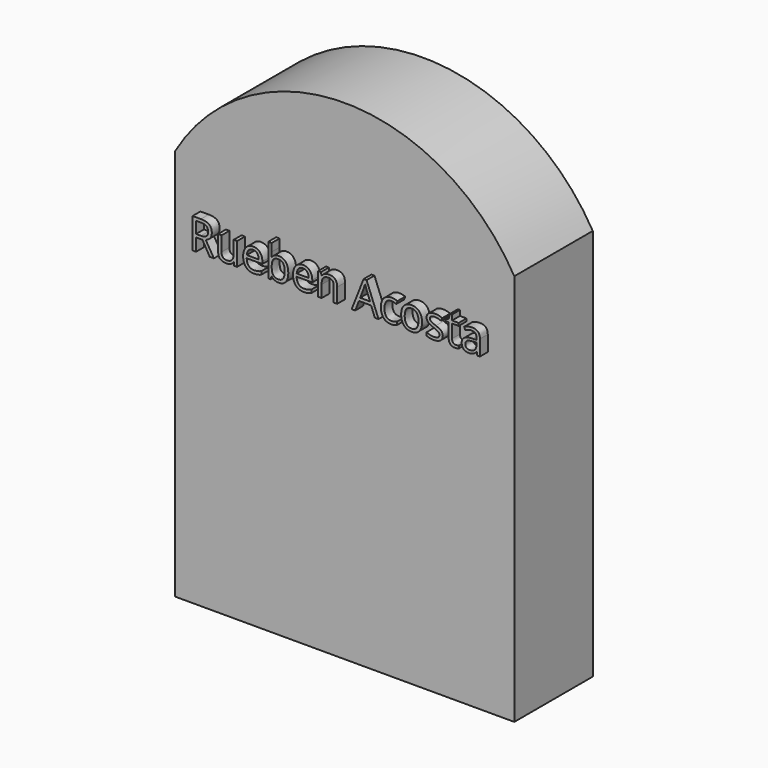
from build123d import *

# Parameters (mm, degrees)
F1_DEPTH     = 12.7
F2_TEXT_SIZE = 5.5030467163
F3_DEPTH     = 1.27


# Not quite as in the source:
# - Text() gives the source's letters only with a copy of the font that has no kerning and outlines rounded to 1/6400 em; it was checked with that copy


with BuildPart() as f1:
    # F0 (on Front) → F1 (new body)
    with BuildSketch(Plane.XZ):
        with BuildLine():
            Line((20.3157289929, -50.8), (20.3157289929, 0))
            ThreePointArc((20.3157289929, 0), (-1.6346000918, 12.6194267313), (-23.5849291764, 0))
            Line((-23.5849291764, 0), (-23.5849291764, -50.8))
            Line((-23.5849291764, -50.8), (20.3157289929, -50.8))
        make_face()
    extrude(amount=-F1_DEPTH)

    # F2 (on Front) → F3 (join)
    with BuildSketch(Plane.XZ):
        with Locations((-20.8640991943, -9.7627924987)):
            Text('Rueben Acosta', F2_TEXT_SIZE, font='Open Sans', text_align=(TextAlign.LEFT, TextAlign.BOTTOM))
    extrude(amount=F3_DEPTH)


solid = f1.part
